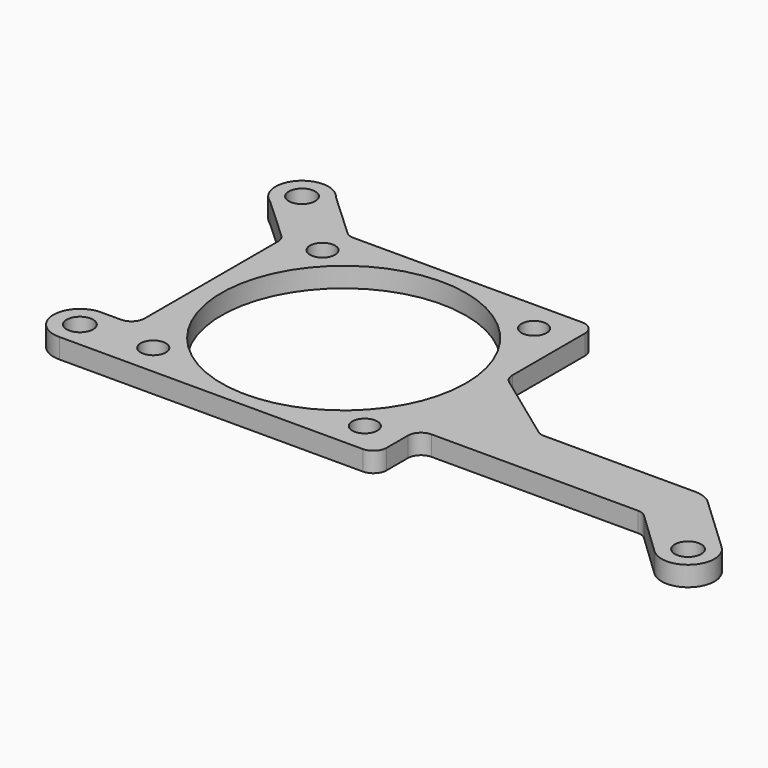
from build123d import *

# Parameters (mm, degrees)
F0_R     = 2
F0_R_2   = 1.9
F0_R_3   = 18.5
F1_DEPTH = 3
F2_R     = 2
F3_R     = 4


with BuildPart() as f1:
    # F0 (on Top) → F1 (new body)
    with BuildSketch(Plane.XY):
        with BuildLine():
            Line((2.0000000052, 16.5001536438), (-35.3637253092, 16.5001536438))
            Line((-35.3637253092, 16.5001536438), (-42.7812429201, 23.375301328))
            ThreePointArc((-42.7812429201, 23.375301328), (-48.9377019653, 23.7146468067), (-48.1133599984, 17.6041964427))
            Line((-48.1133599984, 17.6041964427), (-40.9999999948, 11.0457026558))
            Line((-40.9999999948, 11.0457026558), (-40.9999999948, -17.0001679047))
            Line((-40.9999999948, -17.0001679047), (-45.9997427603, -17.0001679047))
            ThreePointArc((-45.9997427603, -17.0001679047), (-49.9991778461, -21.0673913699), (-45.8653148176, -24.9979084075))
            Line((-45.8653148176, -24.9979084075), (2.0000000052, -24.9998463562))
            Line((2.0000000052, -24.9998463562), (2.0000000052, -16.9998463562))
            Line((2.0000000052, -16.9998463562), (14.0000000052, -16.9998463562))
            Line((14.0000000052, -16.9998463562), (36.0000000052, -16.9998463562))
            Line((36.0000000052, -16.9998463562), (43.2410032397, -23.8966064518))
            ThreePointArc((43.2410032397, -23.8966064518), (48.9041379149, -23.7505294783), (48.7417034391, -18.0878403757))
            Line((48.7417034391, -18.0878403757), (39.0890352428, -8.999838983))
            Line((39.0890352428, -8.999838983), (14.0000000052, -8.999838983))
            Line((14.0000000052, -8.999838983), (2.0000000052, -0.2498463562))
            Line((2.0000000052, -0.2498463562), (2.0000000052, 16.5001536438))
        make_face()
        with Locations((-45.9997427603, -21.0001679047)):
            Circle(F0_R, mode=Mode.SUBTRACT)
        with Locations((-35.5, -20.25)):
            Circle(F0_R_2, mode=Mode.SUBTRACT)
        with Locations((-3.5, -20.25)):
            Circle(F0_R_2, mode=Mode.SUBTRACT)
        with Locations((-19.5, -4.25)):
            Circle(F0_R_3, mode=Mode.SUBTRACT)
        with Locations((45.9997427603, -21.0001679047)):
            Circle(F0_R, mode=Mode.SUBTRACT)
        with Locations((-35.5, 11.75)):
            Circle(F0_R_2, mode=Mode.SUBTRACT)
        with Locations((-3.5, 11.75)):
            Circle(F0_R_2, mode=Mode.SUBTRACT)
        with Locations((-45.9997427603, 21.0001679047)):
            Circle(F0_R, mode=Mode.SUBTRACT)
    extrude(amount=F1_DEPTH)

    # F2
    f2_edges = [f1.edges().sort_by_distance(p)[0] for p in [
        (-41, -17.000168, 1.5),
        (-41, 11.045703, 1.5),
        (-35.363725, 16.500154, 1.5),
        (2, 16.500154, 1.5),
        (2, -16.999846, 1.5),
        (2, -0.249846, 1.5),
        (36, -16.999846, 1.5),
        (2, -24.999846, 1.5),
        (14, -8.999839, 1.5),
    ]]
    fillet(f2_edges, radius=F2_R)

    # F3
    f3_edges = [f1.edges().sort_by_distance(p)[0] for p in [
        (39.089035, -8.999839, 1.5),
    ]]
    fillet(f3_edges, radius=F3_R)


solid = f1.part
